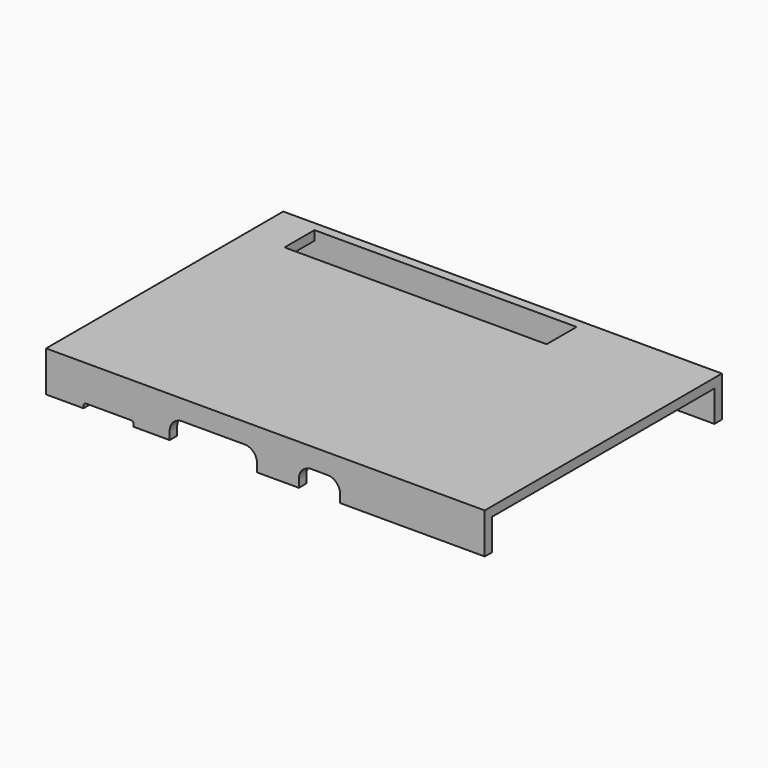
from build123d import *

# Parameters (mm, degrees)
F0_W     = 89.253187
F0_H     = 60.325
F1_DEPTH = 1.905
F3_DEPTH = 6.35
F5_DEPTH = 25.4
F6_W     = 53.34
F6_H     = 7.62
F7_DEPTH = 25.4


# Not quite as in the source:
# - a feature names something its author has since deleted; it is built from what else it names


with BuildPart() as f1:
    # F0 (on Top) → F1 (new body)
    with BuildSketch(Plane.XY):
        Rectangle(F0_W, F0_H)
    extrude(amount=F1_DEPTH)

    # F2 (on face) → F3 (join)
    with BuildSketch(Plane(origin=(0, 0, 0), x_dir=(1, 0, 0), z_dir=(0, 0, -1))):
        Polygon((-42.7215935, -28.2575), (-42.7215935, 28.2575), (44.6265935, 28.2575), (44.6265935, 30.1625), (-44.6265935, 30.1625), (-44.6265935, -30.1625), (44.6265935, -30.1625), (44.6265935, -28.2575), align=None)
    extrude(amount=F3_DEPTH)

    # F4 (on face) → F5 (cut)
    with BuildSketch(Plane.XZ.offset(30.1625)):
        with BuildLine():
            Line((-37.0065935, -5.842), (-37.0065935, -6.35))
            Line((-37.0065935, -6.35), (-26.8465935, -6.35))
            Line((-26.8465935, -6.35), (-26.8465935, -5.842))
            ThreePointArc((-26.8465935, -5.842), (-26.9953832552, -5.4827897552), (-27.3545935, -5.334))
            Line((-27.3545935, -5.334), (-36.4985935, -5.334))
            ThreePointArc((-36.4985935, -5.334), (-36.8578037448, -5.4827897552), (-37.0065935, -5.842))
        make_face()
        with BuildLine():
            Line((-19.4805935, -4.699), (-19.4805935, -6.35))
            Line((-19.4805935, -6.35), (-1.7005935, -6.35))
            Line((-1.7005935, -6.35), (-1.7005935, -4.699))
            ThreePointArc((-1.7005935, -4.699), (-2.4445422758, -2.9029487758), (-4.2405935, -2.159))
            Line((-4.2405935, -2.159), (-16.9405935, -2.159))
            ThreePointArc((-16.9405935, -2.159), (-18.7366447242, -2.9029487758), (-19.4805935, -4.699))
        make_face()
        with BuildLine():
            Line((6.8084065, -4.699), (6.8084065, -6.35))
            Line((6.8084065, -6.35), (15.1904065, -6.35))
            Line((15.1904065, -6.35), (15.1904065, -4.699))
            ThreePointArc((15.1904065, -4.699), (14.4464577242, -2.9029487758), (12.6504065, -2.159))
            Line((12.6504065, -2.159), (9.3484065, -2.159))
            ThreePointArc((9.3484065, -2.159), (7.5523552758, -2.9029487758), (6.8084065, -4.699))
        make_face()
    extrude(amount=-F5_DEPTH, mode=Mode.SUBTRACT)

    # F6 (on face) → F7 (cut)
    with BuildSketch(Plane.XY.offset(1.905)):
        with Locations((-10.0825935, 24.4475)):
            Rectangle(F6_W, F6_H)
    extrude(amount=-F7_DEPTH, mode=Mode.SUBTRACT)


solid = f1.part
